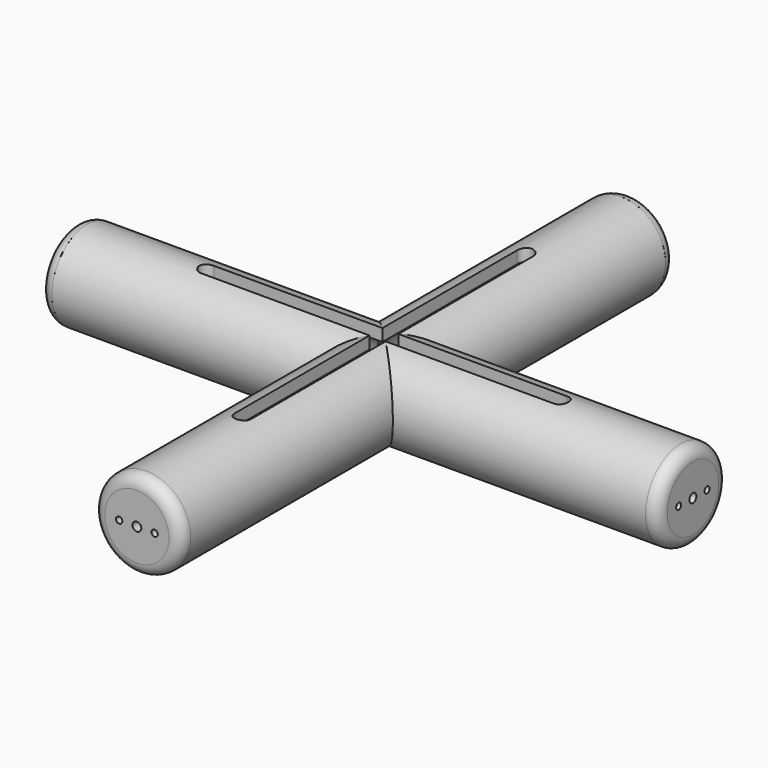
from build123d import *

# Parameters (mm, degrees)
F0_R                   = 69.8
F0_R_2                 = 50.8
F1_DEPTH               = 469.9
F2_R                   = 69.8
F2_R_2                 = 50.8
F3_DEPTH               = 469.9
F4_D                   = 101.6
F4_DEPTH               = 469.9010001
F5_D                   = 101.6
F6_D                   = 101.6
F6_DEPTH               = 469.9010001
F7_D                   = 101.6
F8_W                   = 25.4
F8_H                   = 25.4
F9_DEPTH               = 76.2
F11_R                  = 69.8
F11_R_2                = 50.8
F11_R_3                = 5
F11_R_4                = 7
F14_DEPTH              = 19
F10_R                  = 69.8
F10_R_2                = 50.8
F10_R_3                = 5
F10_R_4                = 7
F15_DEPTH              = 19
F12_R                  = 69.8
F12_R_2                = 50.8
F12_R_3                = 5
F12_R_4                = 7
F16_DEPTH              = 19
F13_R                  = 69.8
F13_R_2                = 50.8
F13_R_3                = 5
F13_R_4                = 7
F17_DEPTH              = 19
F18_R                  = 18.99999
F19_D                  = 8
F19_DEPTH              = 20
F19_CSINK_D            = 25
F19_CSINK_ANGLE        = 100
F19_TIP                = 2.4034424761
F19_ON_F13_D           = 8
F19_ON_F13_DEPTH       = 20
F19_ON_F13_CSINK_D     = 25
F19_ON_F13_CSINK_ANGLE = 100
F19_ON_F13_TIP         = 2.4034424761
F19_ON_F10_D           = 8
F19_ON_F10_DEPTH       = 20
F19_ON_F10_CSINK_D     = 25
F19_ON_F10_CSINK_ANGLE = 100
F19_ON_F10_TIP         = 2.4034424761
F19_ON_F11_D           = 8
F19_ON_F11_DEPTH       = 20
F19_ON_F11_CSINK_D     = 25
F19_ON_F11_CSINK_ANGLE = 100
F19_ON_F11_TIP         = 2.4034424761


# Not quite as in the source:
# - a fillet or chamfer is up to 0.001 mm smaller than in the source, because OpenCascade refuses the exact size


with BuildPart() as f1:
    # F0 (on Front) → F1 (new body, symmetric)
    with BuildSketch(Plane.XZ):
        Circle(F0_R)
        Circle(F0_R_2, mode=Mode.SUBTRACT)
    extrude(amount=F1_DEPTH, both=True)

    # F2 (on Right) → F3 (join, symmetric)
    with BuildSketch(Plane.YZ):
        Circle(F2_R)
        Circle(F2_R_2, mode=Mode.SUBTRACT)
    extrude(amount=F3_DEPTH, both=True)

    # F4 (through all, one way)
    with BuildSketch(Plane(origin=(0, 0, 0), x_dir=(0, 1, 0), z_dir=(-1, 0, 0))):
        with Locations((0, 0)):
            Circle(F4_D / 2)
    extrude(amount=-F4_DEPTH, mode=Mode.SUBTRACT)

    # F5 (through all)
    with Locations(Plane.YZ):
        with Locations((0, 0)):
            Hole(F5_D / 2)

    # F6 (through all, one way)
    with BuildSketch(Plane(origin=(0, 0, 0), x_dir=(1, 0, 0), z_dir=(0, 1, 0))):
        with Locations((0, 0)):
            Circle(F6_D / 2)
    extrude(amount=-F6_DEPTH, mode=Mode.SUBTRACT)

    # F7 (through all)
    with Locations(Plane.XZ):
        with Locations((0, 0)):
            Hole(F7_D / 2)

    # F8 (on Top) → F9 (cut)
    with BuildSketch(Plane.XY):
        with BuildLine():
            Line((-12.7, -12.7), (-12.7, 12.7))
            Line((-12.7, 12.7), (-279.4, 12.7))
            ThreePointArc((-279.4, 12.7), (-292.1, 0), (-279.4, -12.7))
            Line((-279.4, -12.7), (-12.7, -12.7))
        make_face()
        with BuildLine():
            ThreePointArc((12.7, 279.4), (0, 292.1), (-12.7, 279.4))
            Line((-12.7, 279.4), (-12.7, 12.7))
            Line((-12.7, 12.7), (12.7, 12.7))
            Line((12.7, 12.7), (12.7, 279.4))
        make_face()
        with BuildLine():
            Line((279.4, 12.7), (12.7, 12.7))
            Line((12.7, 12.7), (12.7, -12.7))
            Line((12.7, -12.7), (279.4, -12.7))
            ThreePointArc((279.4, -12.7), (292.1, 0), (279.4, 12.7))
        make_face()
        with BuildLine():
            Line((12.7, -12.7), (-12.7, -12.7))
            Line((-12.7, -12.7), (-12.7, -279.4))
            ThreePointArc((-12.7, -279.4), (0, -292.1), (12.7, -279.4))
            Line((12.7, -279.4), (12.7, -12.7))
        make_face()
        Rectangle(F8_W, F8_H)
    extrude(amount=F9_DEPTH, mode=Mode.SUBTRACT)

    # F11 (on face) → F14 (join)
    with BuildSketch(Plane(origin=(0, 469.9, 0), x_dir=(-1, 0, 0), z_dir=(0, 1, 0))):
        Circle(F11_R)
        Circle(F11_R_2, mode=Mode.SUBTRACT)
        Circle(F11_R_2)
        with Locations((-28.077211231, 0)):
            Circle(F11_R_3, mode=Mode.SUBTRACT)
        Circle(F11_R_4, mode=Mode.SUBTRACT)
        with Locations((28.077211231, 0)):
            Circle(F11_R_3, mode=Mode.SUBTRACT)
    extrude(amount=F14_DEPTH)

    # F10 (on face) → F15 (join)
    with BuildSketch(Plane(origin=(-469.9, 0, 0), x_dir=(0, -1, 0), z_dir=(-1, 0, 0))):
        Circle(F10_R)
        Circle(F10_R_2, mode=Mode.SUBTRACT)
        Circle(F10_R_2)
        with Locations((-28.077211231, 0)):
            Circle(F10_R_3, mode=Mode.SUBTRACT)
        Circle(F10_R_4, mode=Mode.SUBTRACT)
        with Locations((28.077211231, 0)):
            Circle(F10_R_3, mode=Mode.SUBTRACT)
    extrude(amount=F15_DEPTH)

    # F12 (on face) → F16 (join)
    with BuildSketch(Plane.YZ.offset(469.9)):
        Circle(F12_R)
        Circle(F12_R_2, mode=Mode.SUBTRACT)
        Circle(F12_R_2)
        with Locations((-28.077211231, 0)):
            Circle(F12_R_3, mode=Mode.SUBTRACT)
        Circle(F12_R_4, mode=Mode.SUBTRACT)
        with Locations((28.077211231, 0)):
            Circle(F12_R_3, mode=Mode.SUBTRACT)
    extrude(amount=F16_DEPTH)

    # F13 (on face) → F17 (join)
    with BuildSketch(Plane.XZ.offset(469.9)):
        Circle(F13_R)
        Circle(F13_R_2, mode=Mode.SUBTRACT)
        Circle(F13_R_2)
        with Locations((-28.077211231, 0)):
            Circle(F13_R_3, mode=Mode.SUBTRACT)
        Circle(F13_R_4, mode=Mode.SUBTRACT)
        with Locations((28.077211231, 0)):
            Circle(F13_R_3, mode=Mode.SUBTRACT)
    extrude(amount=F17_DEPTH)

    # F18 (radius 19 in the source; OpenCascade refuses exactly that, so slightly less here)
    f18_edges = [f1.edges().sort_by_distance(p)[0] for p in [
        (-488.9, 69.8, 0),
        (69.8, 488.9, 0),
        (488.9, -69.8, 0),
        (-69.8, -488.9, 0),
    ]]
    fillet(f18_edges, radius=F18_R)

    # F19
    with Locations(Plane(origin=(469.9, 0, 0), x_dir=(0, 1, 0), z_dir=(-1, 0, 0))):
        with Locations((28.077211231, 0), (-28.077211231, 0)):
            CounterSinkHole(F19_D / 2, F19_CSINK_D / 2, depth=F19_DEPTH, counter_sink_angle=F19_CSINK_ANGLE)
            with Locations((0, 0, -(F19_DEPTH + F19_TIP / 2))):  # 118° drill point
                Cone(0, F19_D / 2, F19_TIP, mode=Mode.SUBTRACT)

    # F19 on F13
    with Locations(Plane(origin=(0, -469.9, 0), x_dir=(1, 0, 0), z_dir=(0, 1, 0))):
        with Locations((-28.077211231, 0), (28.077211231, 0)):
            CounterSinkHole(F19_ON_F13_D / 2, F19_ON_F13_CSINK_D / 2, depth=F19_ON_F13_DEPTH, counter_sink_angle=F19_ON_F13_CSINK_ANGLE)
            with Locations((0, 0, -(F19_ON_F13_DEPTH + F19_ON_F13_TIP / 2))):  # 118° drill point
                Cone(0, F19_ON_F13_D / 2, F19_ON_F13_TIP, mode=Mode.SUBTRACT)

    # F19 on F10
    with Locations(Plane(origin=(-469.9, 0, 0), x_dir=(0, -1, 0), z_dir=(1, 0, 0))):
        with Locations((28.077211231, 0), (-28.077211231, 0)):
            CounterSinkHole(F19_ON_F10_D / 2, F19_ON_F10_CSINK_D / 2, depth=F19_ON_F10_DEPTH, counter_sink_angle=F19_ON_F10_CSINK_ANGLE)
            with Locations((0, 0, -(F19_ON_F10_DEPTH + F19_ON_F10_TIP / 2))):  # 118° drill point
                Cone(0, F19_ON_F10_D / 2, F19_ON_F10_TIP, mode=Mode.SUBTRACT)

    # F19 on F11
    with Locations(Plane(origin=(0, 469.9, 0), x_dir=(-1, 0, 0), z_dir=(0, -1, 0))):
        with Locations((28.077211231, 0), (-28.077211231, 0)):
            CounterSinkHole(F19_ON_F11_D / 2, F19_ON_F11_CSINK_D / 2, depth=F19_ON_F11_DEPTH, counter_sink_angle=F19_ON_F11_CSINK_ANGLE)
            with Locations((0, 0, -(F19_ON_F11_DEPTH + F19_ON_F11_TIP / 2))):  # 118° drill point
                Cone(0, F19_ON_F11_D / 2, F19_ON_F11_TIP, mode=Mode.SUBTRACT)


solid = f1.part
